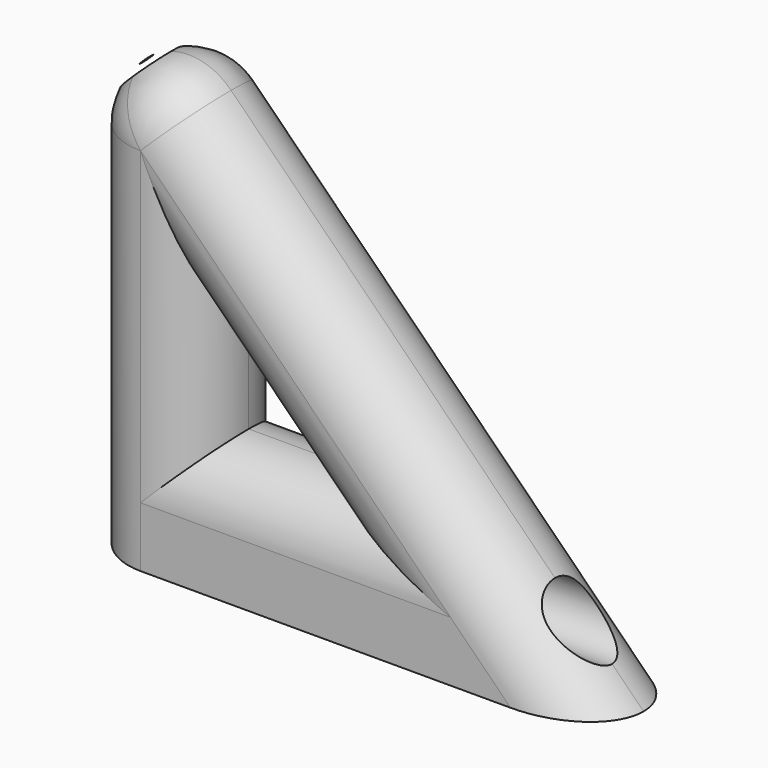
from build123d import *

# Parameters (mm, degrees)
F1_DEPTH = 14
F2_R     = 6.99999
F3_R     = 3.325
F4_DEPTH = 75
F6_R     = 3.325
F7_DEPTH = 45


# Not quite as in the source:
# - a fillet or chamfer is up to 0.001 mm smaller than in the source, because OpenCascade refuses the exact size


with BuildPart() as f1:
    # F0 (on Front) → F1 (new body)
    with BuildSketch(Plane.XZ):
        with BuildLine():
            Line((-60, 0), (0, 0))
            Line((0, 0), (-48.0502525317, 48.0502525317))
            ThreePointArc((-48.0502525317, 48.0502525317), (-52.6133842686, 50.0898203572), (-57.3736269721, 48.5659773311))
            ThreePointArc((-57.3736269721, 48.5659773311), (-59.3093339111, 46.1323865911), (-60, 43.1005050634))
            Line((-60, 43.1005050634), (-60, 0))
        make_face()
        Polygon((-33.7989898732, 14), (-46, 14), (-46, 26.2010101268), align=None, mode=Mode.SUBTRACT)
    extrude(amount=F1_DEPTH)

    # F2 (radius 7 in the source; OpenCascade refuses exactly that, so slightly less here)
    f2_edges = [f1.edges().sort_by_distance(p)[0] for p in [
        (-24.025126, -14, 24.025126),
        (-39.899495, -14, 20.100505),
        (-46, -14, 20.100505),
        (-39.899495, -14, 14),
        (-24.025126, 0, 24.025126),
        (-39.899495, 0, 20.100505),
        (-46, 0, 20.100505),
        (-39.899495, 0, 14),
    ]]
    fillet(f2_edges, radius=F2_R)

    # F3 (on Right) → F4 (cut)
    with BuildSketch(Plane.YZ):
        with Locations((-7, 7)):
            Circle(F3_R)
    extrude(amount=-F4_DEPTH, mode=Mode.SUBTRACT)

    # F6 (on face) → F7 (cut)
    with BuildSketch(Plane(origin=(-52.9698021516, 0, 52.9698021516), x_dir=(0, -1, 0), z_dir=(-0.7071067812, 0, 0.7071067812))):
        with Locations((7, -7)):
            Circle(F6_R)
    extrude(amount=-F7_DEPTH, mode=Mode.SUBTRACT)


solid = f1.part
